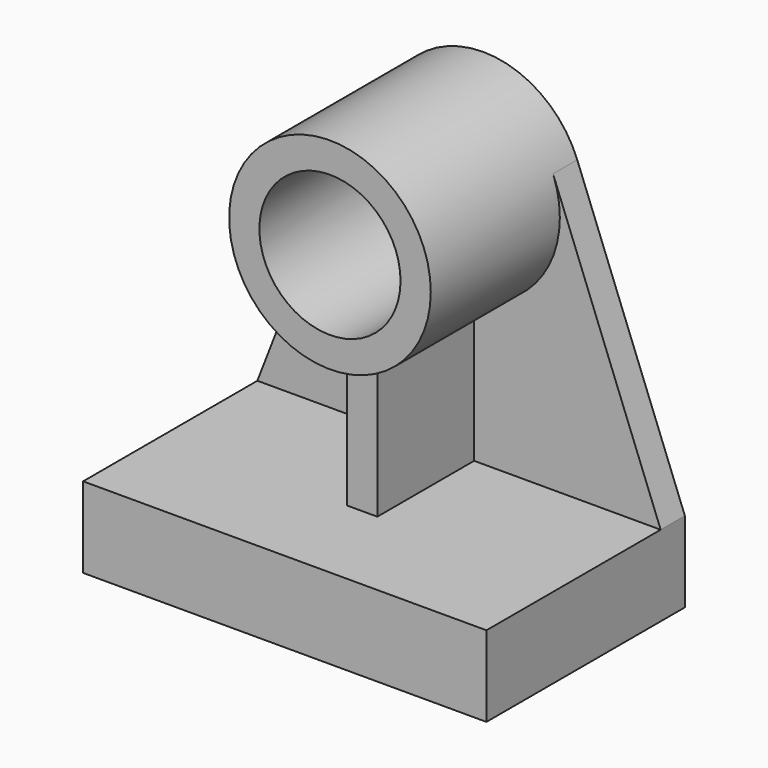
from build123d import *

# Parameters (mm, degrees)
F0_R     = 44.45
F1_DEPTH = 19.05
F2_W     = 254
F2_H     = 50.8
F3_DEPTH = 137.16
F4_R     = 63.5
F4_R_2   = 44.45
F5_DEPTH = 101.6
F6_W     = 19.05
F6_H     = 89.6184392118
F7_DEPTH = 76.2


with BuildPart() as f1:
    # F0 (on Front) → F1 (new body)
    with BuildSketch(Plane.XZ):
        with BuildLine():
            ThreePointArc((-59.2277468166, 22.8981223472), (-11.6466320699, -62.4228000127), (63.5, 0))
            ThreePointArc((63.5, 0), (62.4228000127, 11.6466320699), (59.2277468166, 22.8981223472))
            ThreePointArc((59.2277468166, 22.8981223472), (0, 63.5), (-59.2277468166, 22.8981223472))
        make_face()
        Circle(F0_R, mode=Mode.SUBTRACT)
        with BuildLine():
            ThreePointArc((59.2277468166, 22.8981223472), (62.4228000127, 11.6466320699), (63.5, 0))
            ThreePointArc((63.5, 0), (-11.6466320699, -62.4228000127), (-59.2277468166, 22.8981223472))
            Line((-59.2277468166, 22.8981223472), (-127, -152.4))
            Line((-127, -152.4), (-127, -203.2))
            Line((-127, -203.2), (127, -203.2))
            Line((127, -203.2), (127, -152.4))
            Line((127, -152.4), (59.2277468166, 22.8981223472))
        make_face()
    extrude(amount=F1_DEPTH)

    # F2 (on face) → F3 (join)
    with BuildSketch(Plane.XZ.offset(19.05)):
        with Locations((0, -177.8)):
            Rectangle(F2_W, F2_H)
    extrude(amount=F3_DEPTH)

    # F4 (on face) → F5 (join)
    with BuildSketch(Plane.XZ.offset(19.05)):
        Circle(F4_R)
        Circle(F4_R_2, mode=Mode.SUBTRACT)
    extrude(amount=F5_DEPTH)

    # F6 (on face) → F7 (join)
    with BuildSketch(Plane.XZ.offset(19.05)):
        with Locations((0, -107.5907803941)):
            Rectangle(F6_W, F6_H)
    extrude(amount=F7_DEPTH)


solid = f1.part
